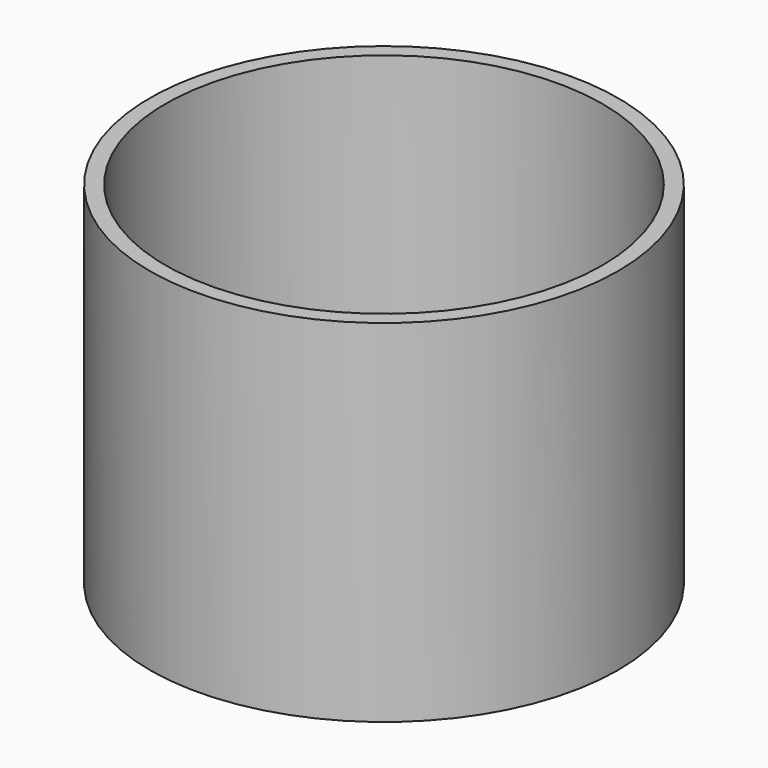
from build123d import *

# Parameters (mm, degrees)
F0_R         = 38.1
F1_DEPTH     = 57.15
F2_T         = -6.096
F3_R         = 35.56
F4_DEPTH     = 53.34
F6_DEPTH     = 2.54
F7_T4_DEPTH  = 21.6761651331
F7_S5_R      = 35.56
F7_T6_DEPTH  = 12
F7_T10_DEPTH = 22.8202736668
F7_S11_R     = 35.56
F7_T12_DEPTH = 13
F7_T16_DEPTH = 29.3439209072
F7_S17_R     = 35.56
F7_T18_DEPTH = 16
F7_T22_DEPTH = 28.6600440275
F7_S23_R     = 35.56
F7_T24_DEPTH = 16
F7_T28_DEPTH = 33.0369286322
F7_S29_R     = 35.56
F7_T30_DEPTH = 18
F7_T34_DEPTH = 33.4811202771
F7_S35_R     = 35.56
F7_T36_DEPTH = 18
F7_T40_DEPTH = 35.8508193235
F7_S41_R     = 35.56
F7_T42_DEPTH = 19
F7_T46_DEPTH = 36.1256776618
F7_S47_R     = 35.56
F7_T48_DEPTH = 20
F7_T52_DEPTH = 37.4813906993
F7_S53_R     = 35.56
F7_T54_DEPTH = 20
F7_T58_DEPTH = 37.6168390252
F7_S59_R     = 35.56
F7_T60_DEPTH = 20
F7_T64_DEPTH = 38.0918347768
F7_S65_R     = 35.56
F7_T66_DEPTH = 21
F7_T70_DEPTH = 38.1
F7_S71_R     = 35.56
F7_T72_DEPTH = 21
F8_COUNT     = 4


# Not quite as in the source:
# - a fillet or chamfer that OpenCascade refuses, or shapes differently, is made with other operations: its cross-section is extruded or revolved along the edge and cut away or added


with BuildPart() as f1:
    # F0 (on Top) → F1 (new body)
    with BuildSketch(Plane.XY):
        Circle(F0_R)
    extrude(amount=F1_DEPTH)

    # F2
    f2_openings = [f1.faces().sort_by_distance(p)[0] for p in [
        (0, 0, 57.15),
    ]]
    offset(amount=F2_T, openings=f2_openings)

    # F3 (on face) → F4 (cut)
    with BuildSketch(Plane.XY.offset(57.15)):
        Circle(F3_R)
    extrude(amount=-F4_DEPTH, mode=Mode.SUBTRACT)

    # F5 (on face) → F6 (join)
    with BuildSketch(Plane.XY.offset(3.81)):
        with BuildLine():
            Line((0, 18.288), (0, 17.526))
            Line((0, 17.526), (30.9411202771, 17.526))
            ThreePointArc((30.9411202771, 17.526), (30.7213870853, 17.9083772451), (30.4969286322, 18.288))
            Line((30.4969286322, 18.288), (0, 18.288))
        make_face()
        with BuildLine():
            Line((26.1200440275, 24.13), (0, 24.13))
            Line((0, 24.13), (0, 23.368))
            Line((0, 23.368), (26.8039209072, 23.368))
            ThreePointArc((26.8039209072, 23.368), (26.4647251469, 23.7514614897), (26.1200440275, 24.13))
        make_face()
        with BuildLine():
            Line((19.1361651331, 29.972), (0, 29.972))
            Line((0, 29.972), (0, 29.21))
            Line((0, 29.21), (20.2802736668, 29.21))
            ThreePointArc((20.2802736668, 29.21), (19.7119018087, 29.5965289702), (19.1361651331, 29.972))
        make_face()
        with BuildLine():
            Line((0, 12.446), (0, 11.684))
            Line((0, 11.684), (33.5856776618, 11.684))
            ThreePointArc((33.5856776618, 11.684), (33.4504183565, 12.065782684), (33.3108193235, 12.446))
            Line((33.3108193235, 12.446), (0, 12.446))
        make_face()
        with BuildLine():
            Line((0, 6.604), (0, 5.842))
            Line((0, 5.842), (35.0768390252, 5.842))
            ThreePointArc((35.0768390252, 5.842), (35.0111879895, 6.2233685061), (34.9413906993, 6.604))
            Line((34.9413906993, 6.604), (0, 6.604))
        make_face()
        with BuildLine():
            Line((0, 0.762), (0, 0))
            Line((0, 0), (35.56, 0))
            ThreePointArc((35.56, 0), (35.5579586356, 0.381021873), (35.5518347768, 0.762))
            Line((35.5518347768, 0.762), (0, 0.762))
        make_face()
    extrude(amount=F6_DEPTH)

    # F7: fillet of radius 0.508 on 12 edges, made by hand


with BuildPart() as f7_tool2:
    # F7_s3 → F7_t4 (new body)
    with BuildSketch(Plane.YZ.offset(20.4061651331)):
        with BuildLine():
            ThreePointArc((29.972, 5.842), (29.8232102448, 6.2012102448), (29.464, 6.35))
            Line((29.464, 6.35), (29.972, 6.35))
            Line((29.972, 6.35), (29.972, 5.842))
        make_face()
    extrude(amount=-F7_T4_DEPTH)

    # F7_s5 → F7_t6 (intersect, symmetric)
    with BuildSketch(Plane.XY.offset(6.1)):
        Circle(F7_S5_R)
    extrude(amount=F7_T6_DEPTH, both=True, mode=Mode.INTERSECT)


with BuildPart() as f1_1:
    add(f1.part)

    # F7_t1: cut F7_tool2
    add(f7_tool2.part, mode=Mode.SUBTRACT)


with BuildPart() as f7_tool8:
    # F7_s9 → F7_t10 (new body)
    with BuildSketch(Plane.YZ.offset(-1.27)):
        with BuildLine():
            ThreePointArc((29.718, 6.35), (29.3587897552, 6.2012102448), (29.21, 5.842))
            Line((29.21, 5.842), (29.21, 6.35))
            Line((29.21, 6.35), (29.718, 6.35))
        make_face()
    extrude(amount=F7_T10_DEPTH)

    # F7_s11 → F7_t12 (intersect, symmetric)
    with BuildSketch(Plane.XY.offset(6.1)):
        Circle(F7_S11_R)
    extrude(amount=F7_T12_DEPTH, both=True, mode=Mode.INTERSECT)


with BuildPart() as f1_2:
    add(f1_1.part)

    # F7_t7: cut F7_tool8
    add(f7_tool8.part, mode=Mode.SUBTRACT)


with BuildPart() as f7_tool14:
    # F7_s15 → F7_t16 (new body)
    with BuildSketch(Plane.YZ.offset(-1.27)):
        with BuildLine():
            ThreePointArc((23.876, 6.35), (23.5167897552, 6.2012102448), (23.368, 5.842))
            Line((23.368, 5.842), (23.368, 6.35))
            Line((23.368, 6.35), (23.876, 6.35))
        make_face()
    extrude(amount=F7_T16_DEPTH)

    # F7_s17 → F7_t18 (intersect, symmetric)
    with BuildSketch(Plane.XY.offset(6.1)):
        Circle(F7_S17_R)
    extrude(amount=F7_T18_DEPTH, both=True, mode=Mode.INTERSECT)


with BuildPart() as f1_3:
    add(f1_2.part)

    # F7_t13: cut F7_tool14
    add(f7_tool14.part, mode=Mode.SUBTRACT)


with BuildPart() as f7_tool20:
    # F7_s21 → F7_t22 (new body)
    with BuildSketch(Plane.YZ.offset(27.3900440275)):
        with BuildLine():
            ThreePointArc((24.13, 5.842), (23.9812102448, 6.2012102448), (23.622, 6.35))
            Line((23.622, 6.35), (24.13, 6.35))
            Line((24.13, 6.35), (24.13, 5.842))
        make_face()
    extrude(amount=-F7_T22_DEPTH)

    # F7_s23 → F7_t24 (intersect, symmetric)
    with BuildSketch(Plane.XY.offset(6.1)):
        Circle(F7_S23_R)
    extrude(amount=F7_T24_DEPTH, both=True, mode=Mode.INTERSECT)


with BuildPart() as f1_4:
    add(f1_3.part)

    # F7_t19: cut F7_tool20
    add(f7_tool20.part, mode=Mode.SUBTRACT)


with BuildPart() as f7_tool26:
    # F7_s27 → F7_t28 (new body)
    with BuildSketch(Plane.YZ.offset(31.7669286322)):
        with BuildLine():
            ThreePointArc((18.288, 5.842), (18.1392102448, 6.2012102448), (17.78, 6.35))
            Line((17.78, 6.35), (18.288, 6.35))
            Line((18.288, 6.35), (18.288, 5.842))
        make_face()
    extrude(amount=-F7_T28_DEPTH)

    # F7_s29 → F7_t30 (intersect, symmetric)
    with BuildSketch(Plane.XY.offset(6.1)):
        Circle(F7_S29_R)
    extrude(amount=F7_T30_DEPTH, both=True, mode=Mode.INTERSECT)


with BuildPart() as f1_5:
    add(f1_4.part)

    # F7_t25: cut F7_tool26
    add(f7_tool26.part, mode=Mode.SUBTRACT)


with BuildPart() as f7_tool32:
    # F7_s33 → F7_t34 (new body)
    with BuildSketch(Plane.YZ.offset(-1.27)):
        with BuildLine():
            ThreePointArc((18.034, 6.35), (17.6747897552, 6.2012102448), (17.526, 5.842))
            Line((17.526, 5.842), (17.526, 6.35))
            Line((17.526, 6.35), (18.034, 6.35))
        make_face()
    extrude(amount=F7_T34_DEPTH)

    # F7_s35 → F7_t36 (intersect, symmetric)
    with BuildSketch(Plane.XY.offset(6.1)):
        Circle(F7_S35_R)
    extrude(amount=F7_T36_DEPTH, both=True, mode=Mode.INTERSECT)


with BuildPart() as f1_6:
    add(f1_5.part)

    # F7_t31: cut F7_tool32
    add(f7_tool32.part, mode=Mode.SUBTRACT)


with BuildPart() as f7_tool38:
    # F7_s39 → F7_t40 (new body)
    with BuildSketch(Plane.YZ.offset(34.5808193235)):
        with BuildLine():
            ThreePointArc((12.446, 5.842), (12.2972102448, 6.2012102448), (11.938, 6.35))
            Line((11.938, 6.35), (12.446, 6.35))
            Line((12.446, 6.35), (12.446, 5.842))
        make_face()
    extrude(amount=-F7_T40_DEPTH)

    # F7_s41 → F7_t42 (intersect, symmetric)
    with BuildSketch(Plane.XY.offset(6.1)):
        Circle(F7_S41_R)
    extrude(amount=F7_T42_DEPTH, both=True, mode=Mode.INTERSECT)


with BuildPart() as f1_7:
    add(f1_6.part)

    # F7_t37: cut F7_tool38
    add(f7_tool38.part, mode=Mode.SUBTRACT)


with BuildPart() as f7_tool44:
    # F7_s45 → F7_t46 (new body)
    with BuildSketch(Plane.YZ.offset(-1.27)):
        with BuildLine():
            ThreePointArc((12.192, 6.35), (11.8327897552, 6.2012102448), (11.684, 5.842))
            Line((11.684, 5.842), (11.684, 6.35))
            Line((11.684, 6.35), (12.192, 6.35))
        make_face()
    extrude(amount=F7_T46_DEPTH)

    # F7_s47 → F7_t48 (intersect, symmetric)
    with BuildSketch(Plane.XY.offset(6.1)):
        Circle(F7_S47_R)
    extrude(amount=F7_T48_DEPTH, both=True, mode=Mode.INTERSECT)


with BuildPart() as f1_8:
    add(f1_7.part)

    # F7_t43: cut F7_tool44
    add(f7_tool44.part, mode=Mode.SUBTRACT)


with BuildPart() as f7_tool50:
    # F7_s51 → F7_t52 (new body)
    with BuildSketch(Plane.YZ.offset(36.2113906993)):
        with BuildLine():
            ThreePointArc((6.604, 5.842), (6.4552102448, 6.2012102448), (6.096, 6.35))
            Line((6.096, 6.35), (6.604, 6.35))
            Line((6.604, 6.35), (6.604, 5.842))
        make_face()
    extrude(amount=-F7_T52_DEPTH)

    # F7_s53 → F7_t54 (intersect, symmetric)
    with BuildSketch(Plane.XY.offset(6.1)):
        Circle(F7_S53_R)
    extrude(amount=F7_T54_DEPTH, both=True, mode=Mode.INTERSECT)


with BuildPart() as f1_9:
    add(f1_8.part)

    # F7_t49: cut F7_tool50
    add(f7_tool50.part, mode=Mode.SUBTRACT)


with BuildPart() as f7_tool56:
    # F7_s57 → F7_t58 (new body)
    with BuildSketch(Plane.YZ.offset(-1.27)):
        with BuildLine():
            ThreePointArc((6.35, 6.35), (5.9907897552, 6.2012102448), (5.842, 5.842))
            Line((5.842, 5.842), (5.842, 6.35))
            Line((5.842, 6.35), (6.35, 6.35))
        make_face()
    extrude(amount=F7_T58_DEPTH)

    # F7_s59 → F7_t60 (intersect, symmetric)
    with BuildSketch(Plane.XY.offset(6.1)):
        Circle(F7_S59_R)
    extrude(amount=F7_T60_DEPTH, both=True, mode=Mode.INTERSECT)


with BuildPart() as f1_10:
    add(f1_9.part)

    # F7_t55: cut F7_tool56
    add(f7_tool56.part, mode=Mode.SUBTRACT)


with BuildPart() as f7_tool62:
    # F7_s63 → F7_t64 (new body)
    with BuildSketch(Plane.YZ.offset(36.8218347768)):
        with BuildLine():
            ThreePointArc((0.762, 5.842), (0.6132102448, 6.2012102448), (0.254, 6.35))
            Line((0.254, 6.35), (0.762, 6.35))
            Line((0.762, 6.35), (0.762, 5.842))
        make_face()
    extrude(amount=-F7_T64_DEPTH)

    # F7_s65 → F7_t66 (intersect, symmetric)
    with BuildSketch(Plane.XY.offset(6.1)):
        Circle(F7_S65_R)
    extrude(amount=F7_T66_DEPTH, both=True, mode=Mode.INTERSECT)


with BuildPart() as f1_11:
    add(f1_10.part)

    # F7_t61: cut F7_tool62
    add(f7_tool62.part, mode=Mode.SUBTRACT)


with BuildPart() as f7_tool68:
    # F7_s69 → F7_t70 (new body)
    with BuildSketch(Plane.YZ.offset(-1.27)):
        with BuildLine():
            ThreePointArc((0, 5.842), (0.1487897552, 6.2012102448), (0.508, 6.35))
            Line((0.508, 6.35), (0, 6.35))
            Line((0, 6.35), (0, 5.842))
        make_face()
    extrude(amount=F7_T70_DEPTH)

    # F7_s71 → F7_t72 (intersect, symmetric)
    with BuildSketch(Plane.XY.offset(6.1)):
        Circle(F7_S71_R)
    extrude(amount=F7_T72_DEPTH, both=True, mode=Mode.INTERSECT)


with BuildPart() as f1_12:
    add(f1_11.part)

    # F7_t67: cut F7_tool68
    add(f7_tool68.part, mode=Mode.SUBTRACT)

    # F8: F1 ×4 about axis
    f8_axis = Axis((0, 0, 3.81), (0, 0, 1))


with BuildPart() as f1_13:
    add(f1_12.part)
    for i in range(1, F8_COUNT):
        add(f1_12.part.rotate(f8_axis, i * 360 / F8_COUNT))


solid = f1_13.part
